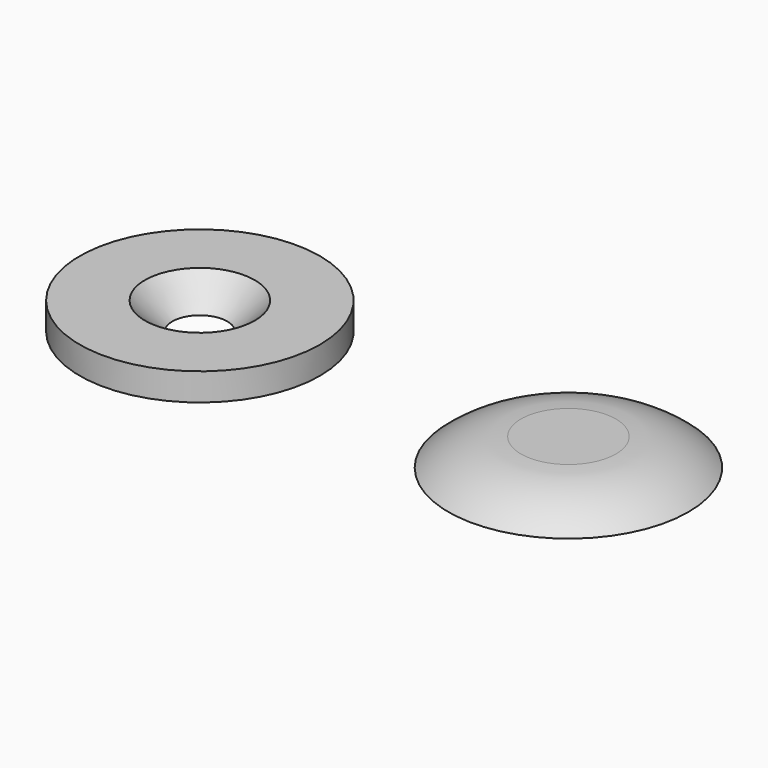
from build123d import *

# Parameters (mm, degrees)
F0_R     = 8.75
F0_R_2   = 2
F1_DEPTH = 2
F2_SIZE  = 1.99999
F3_DEPTH = 2


# Not quite as in the source:
# - a fillet or chamfer that OpenCascade refuses, or shapes differently, is made with other operations: its cross-section is extruded or revolved along the edge and cut away or added
# - a fillet or chamfer is up to 0.001 mm smaller than in the source, because OpenCascade refuses the exact size


with BuildPart() as f1:
    # F0 (on Top) → F1 (new body)
    with BuildSketch(Plane.XY):
        Circle(F0_R)
        Circle(F0_R_2, mode=Mode.SUBTRACT)
    extrude(amount=F1_DEPTH)

    # F2 (size 2 in the source; OpenCascade refuses exactly that, so slightly less here)
    f2_edges = [f1.edges().sort_by_distance(p)[0] for p in [
        (-2, 0, 2),
    ]]
    chamfer(f2_edges, length=F2_SIZE)


with BuildPart() as f3:
    # F0 (on Top) → F3 (new body)
    with BuildSketch(Plane.XY):
        with Locations((26.8592014909, 0)):
            Circle(F0_R)
    extrude(amount=F3_DEPTH)

    # F4: fillet of radius 8 on 1 edges, made by hand

    # F4_s1 → F4_t2 (revolve, cut)
    with BuildSketch(Plane.XZ):
        with BuildLine():
            ThreePointArc((35.6092014909, 0), (33.1461259935, 1.4833147735), (30.3176988687, 2))
            Line((30.3176988687, 2), (30.3176988687, 2.16))
            Line((30.3176988687, 2.16), (35.6092014909, 2.16))
            Line((35.6092014909, 2.16), (35.7692014909, 2))
            ThreePointArc((35.7692014909, 2), (35.7692014909, 1), (35.7150315433, 0.12))
            Line((35.7150315433, 0.12), (35.6092014909, 0))
        make_face()
    revolve(axis=Axis((26.8592014909, 0, 2), (0, 0, 1)), mode=Mode.SUBTRACT)


solid = Compound([f1.part, f3.part])
